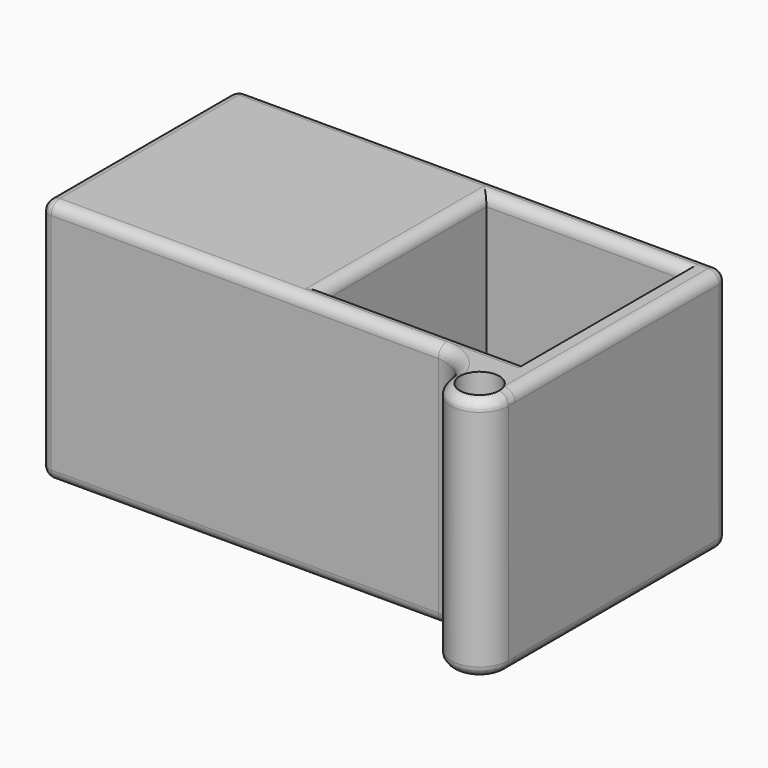
from build123d import *

# Parameters (mm, degrees)
F1_DEPTH              = 34.2
F2_W                  = 28.2
F2_H                  = 28.2
F3_DEPTH              = 31.2
F4_W                  = 34.2
F4_H                  = 34.2
F5_DEPTH              = 34.2
F6_W                  = 28.2
F6_H                  = 28.2
F7_DEPTH              = 31.2
F10_D                 = 3.3
F10_DEPTH             = 25
F10_CSINK_D           = 6.72
F10_CSINK_ANGLE       = 90
F10_TIP               = 0.9914200214
F10_ON_F9_D           = 3.3
F10_ON_F9_DEPTH       = 25
F10_ON_F9_CSINK_D     = 6.72
F10_ON_F9_CSINK_ANGLE = 90
F10_ON_F9_TIP         = 0.9914200214
F12_D                 = 5.5
F13_R                 = 5
F14_R                 = 1.49999


# Not quite as in the source:
# - a fillet or chamfer is up to 0.001 mm smaller than in the source, because OpenCascade refuses the exact size


with BuildPart() as f1:
    # F0 (on Top) → F1 (new body)
    with BuildSketch(Plane.XY):
        Polygon((-34.2, 0), (-8, 0), (0, 0), (0, 34.2), (-34.2, 34.2), align=None)
        with BuildLine():
            Line((0, 0), (-8, 0))
            Line((-8, 0), (-8, -4))
            ThreePointArc((-8, -4), (-4, -8), (0, -4))
            Line((0, -4), (0, 0))
        make_face()
    extrude(amount=F1_DEPTH)

    # F2 (on face) → F3 (cut)
    with BuildSketch(Plane.XY.offset(34.2)):
        with Locations((-17.1, 17.1)):
            Rectangle(F2_W, F2_H)
    extrude(amount=-F3_DEPTH, mode=Mode.SUBTRACT)

    # F4 (on face) → F5 (join)
    with BuildSketch(Plane(origin=(-34.2, 0, 0), x_dir=(0, -1, 0), z_dir=(-1, 0, 0))):
        with Locations((-17.1, 17.1)):
            Rectangle(F4_W, F4_H)
    extrude(amount=F5_DEPTH)

    # F6 (on face) → F7 (cut)
    with BuildSketch(Plane(origin=(-68.4, 0, 0), x_dir=(0, -1, 0), z_dir=(-1, 0, 0))):
        with Locations((-17.1, 17.1)):
            Rectangle(F6_W, F6_H)
    extrude(amount=-F7_DEPTH, mode=Mode.SUBTRACT)

    # F10
    with Locations(Plane(origin=(0, 34.2, 0), x_dir=(-1, 0, 0), z_dir=(0, 1, 0))):
        with Locations((17.05, 17.1), (51.35, 17.1)):
            CounterSinkHole(F10_D / 2, F10_CSINK_D / 2, depth=F10_DEPTH, counter_sink_angle=F10_CSINK_ANGLE)
            with Locations((0, 0, -(F10_DEPTH + F10_TIP / 2))):  # 118° drill point
                Cone(0, F10_D / 2, F10_TIP, mode=Mode.SUBTRACT)

    # F10 on F9
    with Locations(Plane(origin=(-37.2, 0, 0), x_dir=(0, -1, 0), z_dir=(-1, 0, 0))):
        with Locations((-17.1, 17.1)):
            CounterSinkHole(F10_ON_F9_D / 2, F10_ON_F9_CSINK_D / 2, depth=F10_ON_F9_DEPTH, counter_sink_angle=F10_ON_F9_CSINK_ANGLE)
            with Locations((0, 0, -(F10_ON_F9_DEPTH + F10_ON_F9_TIP / 2))):  # 118° drill point
                Cone(0, F10_ON_F9_D / 2, F10_ON_F9_TIP, mode=Mode.SUBTRACT)

    # F12 (through all)
    with Locations(Plane.XY.offset(34.2)):
        with Locations((-4, -4)):
            Hole(F12_D / 2)

    # F13
    f13_edges = [f1.edges().sort_by_distance(p)[0] for p in [
        (-8, 0, 17.1),
    ]]
    fillet(f13_edges, radius=F13_R)

    # F14 (radius 1.5 in the source; OpenCascade refuses exactly that, so slightly less here)
    f14_edges = [f1.edges().sort_by_distance(p)[0] for p in [
        (-17.1, 3, 34.2),
        (-31.2, 17.1, 34.2),
        (-17.1, 31.2, 34.2),
        (-17.1, 31.2, 3),
        (0, 15.1, 34.2),
        (-40.672136, 0, 34.2),
        (-68.4, 17.1, 34.2),
        (-34.2, 34.2, 34.2),
        (0, 34.2, 17.1),
        (-68.4, 17.1, 31.2),
        (-68.4, 0, 17.1),
        (-68.4, 3, 17.1),
        (-68.4, 31.2, 17.1),
        (-68.4, 34.2, 17.1),
        (-68.4, 17.1, 3),
        (-68.4, 17.1, 0),
        (-40.672136, 0, 0),
        (-34.2, 34.2, 0),
    ]]
    fillet(f14_edges, radius=F14_R)


solid = f1.part
